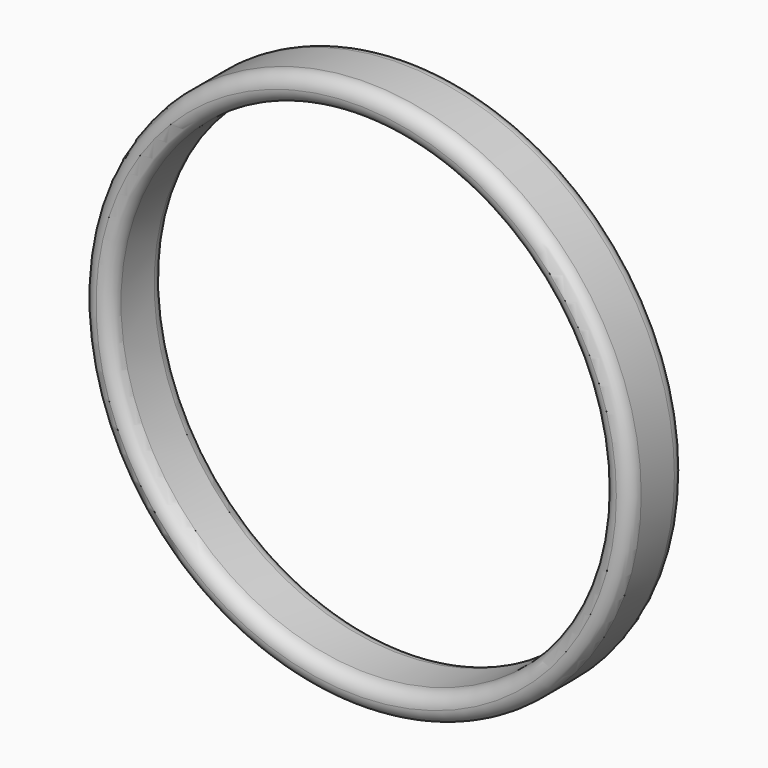
from build123d import *

# Parameters (mm, degrees)
F0_R     = 10.0711
F0_R_2   = 9.0551
F1_DEPTH = 1.27
F2_R     = 0.50799


# Not quite as in the source:
# - a fillet or chamfer is up to 0.001 mm smaller than in the source, because OpenCascade refuses the exact size


with BuildPart() as f1:
    # F0 (on Front) → F1 (new body, symmetric)
    with BuildSketch(Plane.XZ):
        Circle(F0_R)
        Circle(F0_R_2, mode=Mode.SUBTRACT)
    extrude(amount=F1_DEPTH, both=True)

    # F2 (radius 0.508 in the source; OpenCascade refuses exactly that, so slightly less here)
    f2_edges = [f1.edges().sort_by_distance(p)[0] for p in [
        (-9.0551, -1.27, 0),
        (-9.0551, 1.27, 0),
        (-10.0711, -1.27, 0),
        (-10.0711, 1.27, 0),
        (10.0711, 0, 0),
    ]]
    fillet(f2_edges, radius=F2_R)


solid = f1.part
